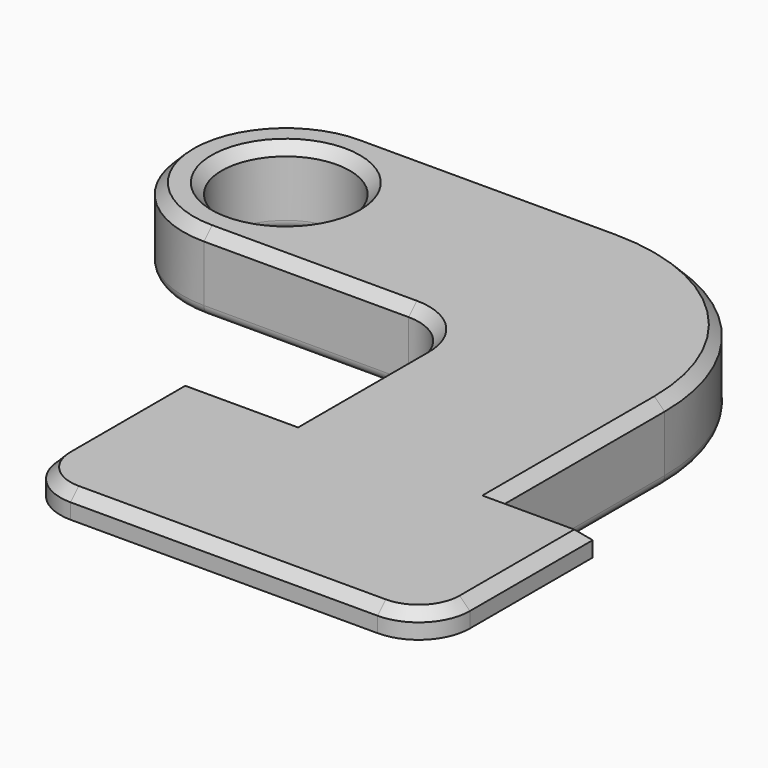
from build123d import *

# Parameters (mm, degrees)
F0_R     = 6.25
F1_DEPTH = 7.5
F2_DEPTH = 2.5
F3_R     = 1
F4_SIZE  = 1


with BuildPart() as f1:
    # F0 (on Top) → F1 (new body)
    with BuildSketch(Plane.XY):
        with BuildLine():
            Line((-15.2574911714, 10), (-40.2574911714, 10))
            ThreePointArc((-40.2574911714, 10), (-50.2574911714, 0), (-40.2574911714, -10))
            Line((-40.2574911714, -10), (-20.2574911714, -10))
            ThreePointArc((-20.2574911714, -10), (-16.7219572654, -11.4644660941), (-15.2574911714, -15))
            Line((-15.2574911714, -15), (-15.2574911714, -30.0000000031))
            Line((-15.2574911714, -30.0000000031), (4.7425088286, -30.0000000031))
            Line((4.7425088286, -30.0000000031), (4.7425088286, -10))
            ThreePointArc((4.7425088286, -10), (-1.1153555476, 4.1421356237), (-15.2574911714, 10))
        make_face()
        with Locations((-40.2574911714, 0)):
            Circle(F0_R, mode=Mode.SUBTRACT)
    extrude(amount=-F1_DEPTH)

    # F0 (on Top) → F2 (join)
    with BuildSketch(Plane.XY):
        with BuildLine():
            Line((13.7208224833, -30.0000000031), (4.7425088286, -30.0000000031))
            Line((4.7425088286, -30.0000000031), (-15.2574911714, -30.0000000031))
            Line((-15.2574911714, -30.0000000031), (-26.2791775167, -30.0000000031))
            Line((-26.2791775167, -30.0000000031), (-26.2791775167, -45.0000000031))
            ThreePointArc((-26.2791775167, -45.0000000031), (-24.8147114226, -48.535533909), (-21.2791775167, -50.0000000031))
            Line((-21.2791775167, -50.0000000031), (8.7208224833, -50.0000000031))
            ThreePointArc((8.7208224833, -50.0000000031), (12.2563563892, -48.535533909), (13.7208224833, -45.0000000031))
            Line((13.7208224833, -45.0000000031), (13.7208224833, -30.0000000031))
        make_face()
    extrude(amount=-F2_DEPTH)

    # F3
    f3_edges = [f1.edges().sort_by_distance(p)[0] for p in [
        (-46.507491, 0, -7.5),
        (-27.757491, 10, -7.5),
        (-50.257491, 0, -7.5),
        (-30.257491, -10, -7.5),
        (-16.721957, -11.464466, -7.5),
        (-15.257491, -22.5, -7.5),
        (-5.257491, -30, -7.5),
        (4.742509, -20, -7.5),
        (-1.115356, 4.142136, -7.5),
        (-5.257491, -30, -2.5),
    ]]
    fillet(f3_edges, radius=F3_R)

    # F4
    f4_edges = [f1.edges().sort_by_distance(p)[0] for p in [
        (-27.757491, 10, 0),
        (-50.257491, 0, 0),
        (-30.257491, -10, 0),
        (-16.721957, -11.464466, 0),
        (-15.257491, -22.5, 0),
        (-20.768334, -30, 0),
        (-26.279178, -37.5, 0),
        (-24.814711, -48.535534, 0),
        (-6.279178, -50, 0),
        (12.256356, -48.535534, 0),
        (13.720822, -37.5, 0),
        (9.231666, -30, 0),
        (4.742509, -20, 0),
        (-1.115356, 4.142136, 0),
        (-46.507491, 0, 0),
    ]]
    chamfer(f4_edges, length=F4_SIZE)


solid = f1.part
